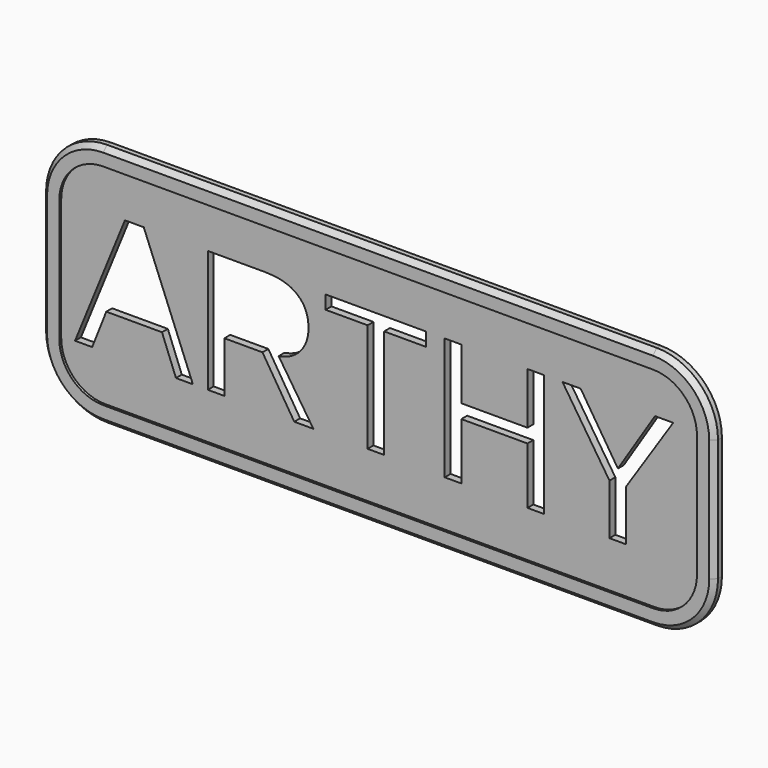
from build123d import *

# Parameters (mm, degrees)
F0_W         = 110
F0_H         = 40
F1_DEPTH     = 1.6
F2_TEXT_SIZE = 29.0988451396
F3_DEPTH     = 1.601
F4_R         = 10
F5_SIZE      = 0.8
F7_DEPTH     = 0.4
F8_DEPTH     = 25
F9_DEPTH     = 25


# Not quite as in the source:
# - Text() gives the source's letters only with a copy of the font that has no kerning and outlines rounded to 1/6400 em; it was checked with that copy


with BuildPart() as f1:
    # F0 (on Front) → F1 (new body)
    with BuildSketch(Plane.XZ):
        Rectangle(F0_W, F0_H)
    extrude(amount=F1_DEPTH)

    # F2 (on face) → F3 (cut, through all)
    with BuildSketch(Plane.XZ.offset(1.6)):
        with Locations((-50, -9.6832554211)):
            Text('ARTHY', F2_TEXT_SIZE, font='Arimo', text_align=(TextAlign.LEFT, TextAlign.BOTTOM))
    extrude(amount=-F3_DEPTH, mode=Mode.SUBTRACT)

    # F4
    f4_edges = [f1.edges().sort_by_distance(p)[0] for p in [
        (55, -0.8, -20),
        (55, -0.8, 20),
        (-55, -0.8, -20),
        (-55, -0.8, 20),
    ]]
    fillet(f4_edges, radius=F4_R)

    # F5
    f5_edges = [f1.edges().sort_by_distance(p)[0] for p in [
        (0, -1.6, -20),
    ]]
    chamfer(f5_edges, length=F5_SIZE)

    # F6 (on face) → F7 (cut)
    with BuildSketch(Plane.XZ.offset(1.6)):
        with BuildLine():
            ThreePointArc((-52.2, -10), (-50.0911688245, -15.0911688245), (-45, -17.2))
            Line((-45, -17.2), (45, -17.2))
            ThreePointArc((45, -17.2), (50.0911688245, -15.0911688245), (52.2, -10))
            Line((52.2, -10), (52.2, 10))
            ThreePointArc((52.2, 10), (50.0911688245, 15.0911688245), (45, 17.2))
            Line((45, 17.2), (-45, 17.2))
            ThreePointArc((-45, 17.2), (-50.0911688245, 15.0911688245), (-52.2, 10))
            Line((-52.2, 10), (-52.2, -10))
        make_face()
    extrude(amount=-F7_DEPTH, mode=Mode.SUBTRACT)

    # F8 (cut): a face of the model
    f8_faces = [f1.faces().sort_by_distance(p)[0] for p in [
        (-40.2608835259, -1.2, 1.5433456147),
    ]]
    extrude(f8_faces, amount=-F8_DEPTH, mode=Mode.SUBTRACT)

    # F9 (cut): a face of the model
    f9_faces = [f1.faces().sort_by_distance(p)[0] for p in [
        (-20.3283992287, -1.2, 4.4737626017),
    ]]
    extrude(f9_faces, amount=-F9_DEPTH, mode=Mode.SUBTRACT)


solid = f1.part
